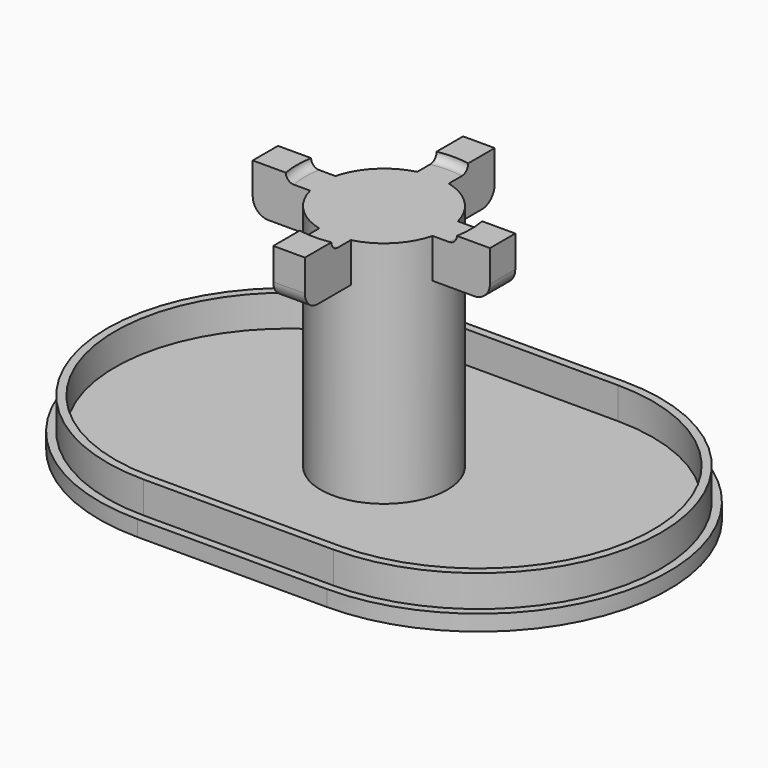
from build123d import *

# Parameters (mm, degrees)
F0_W      = 609.6
F0_H      = 25.4
F0_H_2    = 1117.6
F0_R      = 203.2
F1_DEPTH  = 50.8
F2_DEPTH  = 101.6
F3_DEPTH  = 762
F4_W      = 101.6
F4_H      = 152.4
F5_DEPTH  = 381
F6_W      = 101.6
F6_H      = 152.4
F7_DEPTH  = 381
F8_R      = 50.8
F9_R      = 279.4
F10_DEPTH = 25.4
F11_R     = 25.39999


# Not quite as in the source:
# - a fillet or chamfer is up to 0.001 mm smaller than in the source, because OpenCascade refuses the exact size


with BuildPart() as f1:
    # F0 (on Top) → F1 (new body)
    with BuildSketch(Plane.XY):
        with BuildLine():
            Line((-304.8, 584.2), (-304.8, 609.6))
            ThreePointArc((-304.8, 609.6), (-914.4, 0), (-304.8, -609.6))
            Line((-304.8, -609.6), (-304.8, -584.2))
            ThreePointArc((-304.8, -584.2), (-889, 0), (-304.8, 584.2))
        make_face()
        with BuildLine():
            Line((-304.8, 558.8), (-304.8, 584.2))
            ThreePointArc((-304.8, 584.2), (-889, 0), (-304.8, -584.2))
            Line((-304.8, -584.2), (-304.8, -558.8))
            ThreePointArc((-304.8, -558.8), (-863.6, 0), (-304.8, 558.8))
        make_face()
        with Locations((0, 596.9)):
            Rectangle(F0_W, F0_H)
        with BuildLine():
            ThreePointArc((304.8, -609.6), (914.4, 0), (304.8, 609.6))
            Line((304.8, 609.6), (304.8, 584.2))
            ThreePointArc((304.8, 584.2), (889, 0), (304.8, -584.2))
            Line((304.8, -584.2), (304.8, -609.6))
        make_face()
        with BuildLine():
            ThreePointArc((304.8, -584.2), (889, 0), (304.8, 584.2))
            Line((304.8, 584.2), (304.8, 558.8))
            ThreePointArc((304.8, 558.8), (863.6, 0), (304.8, -558.8))
            Line((304.8, -558.8), (304.8, -584.2))
        make_face()
        with Locations((0, -596.9)):
            Rectangle(F0_W, F0_H)
        with Locations((0, -571.5)):
            Rectangle(F0_W, F0_H)
        Rectangle(F0_W, F0_H_2)
        Circle(F0_R, mode=Mode.SUBTRACT)
        with BuildLine():
            ThreePointArc((304.8, -558.8), (863.6, 0), (304.8, 558.8))
            Line((304.8, 558.8), (304.8, -558.8))
        make_face()
        with BuildLine():
            Line((-304.8, -558.8), (-304.8, 558.8))
            ThreePointArc((-304.8, 558.8), (-863.6, 0), (-304.8, -558.8))
        make_face()
        with Locations((0, 571.5)):
            Rectangle(F0_W, F0_H)
        Circle(F0_R)
    extrude(amount=-F1_DEPTH)

    # F0 (on Top) → F2 (join)
    with BuildSketch(Plane.XY):
        with BuildLine():
            Line((-304.8, 558.8), (-304.8, 584.2))
            ThreePointArc((-304.8, 584.2), (-889, 0), (-304.8, -584.2))
            Line((-304.8, -584.2), (-304.8, -558.8))
            ThreePointArc((-304.8, -558.8), (-863.6, 0), (-304.8, 558.8))
        make_face()
        with Locations((0, -571.5)):
            Rectangle(F0_W, F0_H)
        with Locations((0, 571.5)):
            Rectangle(F0_W, F0_H)
        with BuildLine():
            ThreePointArc((304.8, -584.2), (889, 0), (304.8, 584.2))
            Line((304.8, 584.2), (304.8, 558.8))
            ThreePointArc((304.8, 558.8), (863.6, 0), (304.8, -558.8))
            Line((304.8, -558.8), (304.8, -584.2))
        make_face()
    extrude(amount=F2_DEPTH)

    # F0 (on Top) → F3 (join)
    with BuildSketch(Plane.XY):
        Circle(F0_R)
    extrude(amount=F3_DEPTH)

    # F4 (on Front) → F5 (join, symmetric)
    with BuildSketch(Plane.XZ):
        with Locations((0, 685.8)):
            Rectangle(F4_W, F4_H)
    extrude(amount=F5_DEPTH, both=True)

    # F6 (on Right) → F7 (join, symmetric)
    with BuildSketch(Plane.YZ):
        with Locations((0, 685.8)):
            Rectangle(F6_W, F6_H)
    extrude(amount=F7_DEPTH, both=True)

    # F8
    f8_edges = [f1.edges().sort_by_distance(p)[0] for p in [
        (0, -381, 609.6),
        (-381, 0, 609.6),
        (0, 381, 609.6),
        (381, 0, 609.6),
    ]]
    fillet(f8_edges, radius=F8_R)

    # F9 (on face) → F10 (cut)
    with BuildSketch(Plane.XY.offset(762)):
        Circle(F9_R)
    extrude(amount=-F10_DEPTH, mode=Mode.SUBTRACT)

    # F11 (radius 25.4 in the source; OpenCascade refuses exactly that, so slightly less here)
    f11_edges = [f1.edges().sort_by_distance(p)[0] for p in [
        (279.4, 0, 736.6),
        (-279.4, 0, 736.6),
        (0, 279.4, 736.6),
        (0, -279.4, 736.6),
    ]]
    fillet(f11_edges, radius=F11_R)


solid = f1.part
